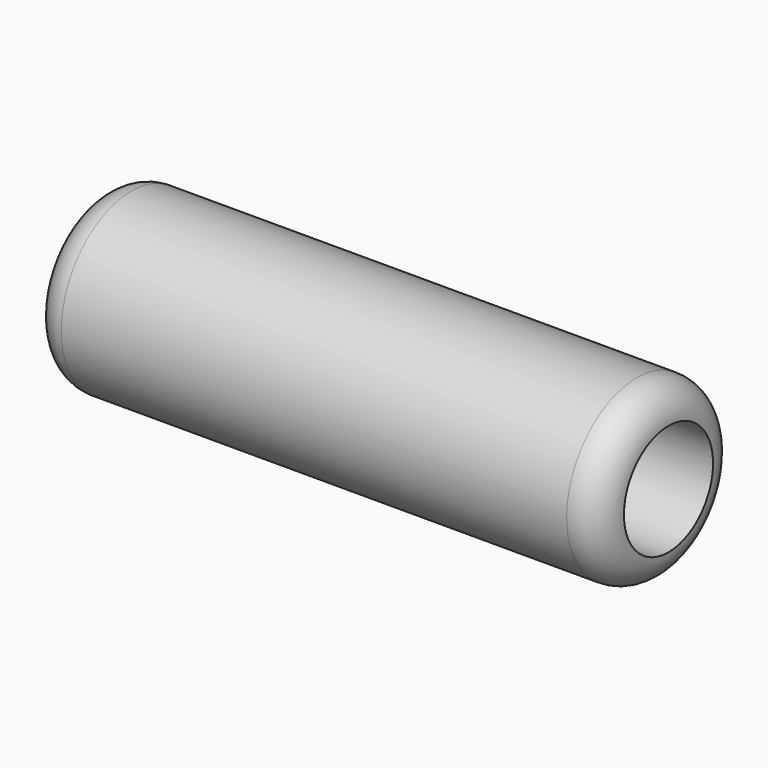
from build123d import *

# Parameters (mm, degrees)
F2_R = 6.34999


# Not quite as in the source:
# - a fillet or chamfer is up to 0.001 mm smaller than in the source, because OpenCascade refuses the exact size


with BuildPart() as f1:
    # F0 (on Front) → F1 (revolve)
    with BuildSketch(Plane.XZ):
        Polygon((3.9624, -4.7625), (0, -4.7625), (0, -17.4625), (113.5126, -17.4625), (113.5126, -11.1125), (3.9624, -11.1125), align=None)
    revolve(axis=Axis((63.5, 0, 0), (1, 0, 0)))

    # F2 (radius 6.35 in the source; OpenCascade refuses exactly that, so slightly less here)
    f2_edges = [f1.edges().sort_by_distance(p)[0] for p in [
        (0, 0, 17.4625),
        (113.5126, 0, 17.4625),
    ]]
    fillet(f2_edges, radius=F2_R)


solid = f1.part
